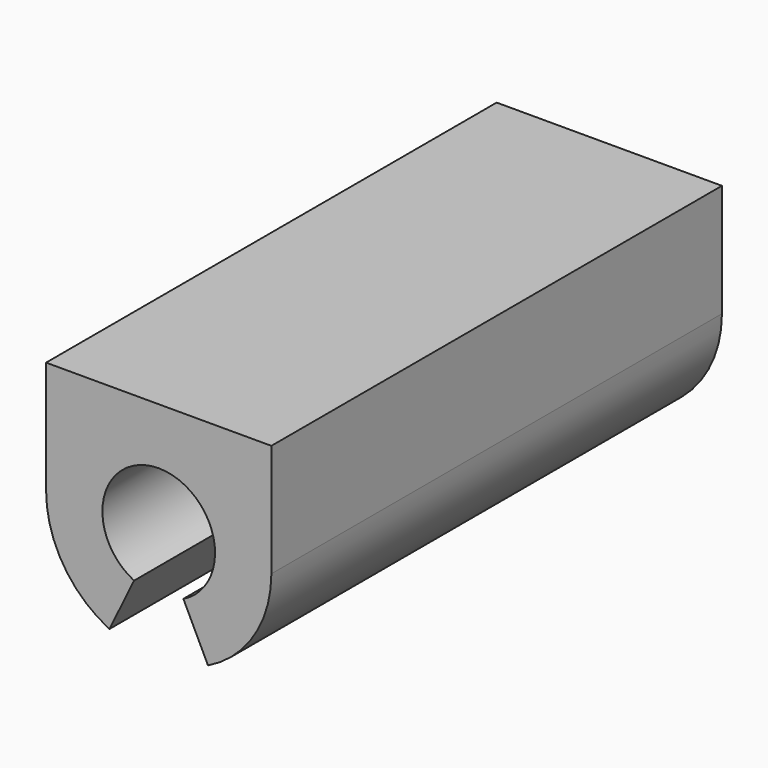
from build123d import *

# Parameters (mm, degrees)
F0_R     = 1
F1_DEPTH = 5
F3_DEPTH = 10.001


# Not quite as in the source:
# - a feature of the source that left no trace in its solid (it failed there, or was rolled back) is left out


with BuildPart() as f1:
    # F0 (on Front) → F1 (new body, symmetric)
    with BuildSketch(Plane.XZ):
        with BuildLine():
            Line((-2, 2), (-2, 0))
            ThreePointArc((-2, 0), (0, -2), (2, 0))
            Line((2, 0), (2, 2))
            Line((2, 2), (0, 2))
            Line((0, 2), (-2, 2))
        make_face()
        Circle(F0_R, mode=Mode.SUBTRACT)
    extrude(amount=F1_DEPTH, both=True)

    # F2 (on face) → F3 (cut, through all)
    with BuildSketch(Plane.XZ.offset(5)):
        with BuildLine():
            Line((0.875, -1.7984368212), (0, 0))
            Line((0, 0), (-0.875, -1.7984368212))
            ThreePointArc((-0.875, -1.7984368212), (0, -2), (0.875, -1.7984368212))
        make_face()
    extrude(amount=-F3_DEPTH, mode=Mode.SUBTRACT)


solid = f1.part
